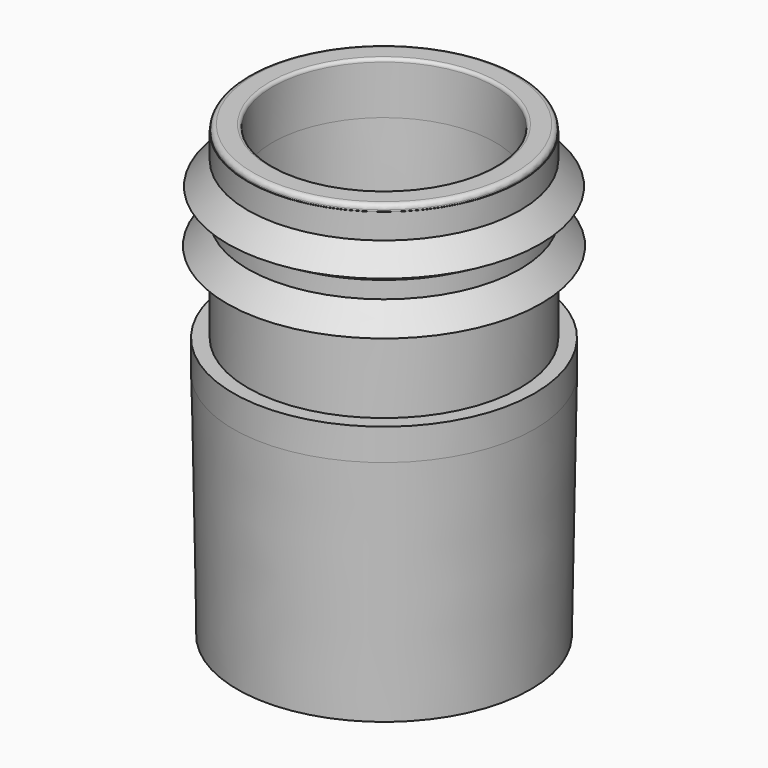
from build123d import *

# Parameters (mm, degrees)
F4_DEPTH      = 9.9510698867
F4_DEPTH_BACK = 9.9510698867


# Not quite as in the source:
# - ends of sketch curves that miss each other by under 0.0002 mm in the source are joined


with BuildPart() as f2:
    # F1 (on Front) → F2 (revolve)
    with BuildSketch(Plane.XZ):
        with BuildLine():
            Line((-0.756877, 0.003809), (-0.990799, 11.890078))
            add(Edge.make_bspline(
                [(-0.990799, 11.890078), (-0.996484, 12.183944), (-1.033002, 12.476088), (-1.099664, 12.762376)],
                knots=[0, 0, 0, 0, 1, 1, 1, 1], degree=3))
            add(Edge.make_bspline(
                [(-1.099664, 12.762376), (-1.116201, 12.833345), (-1.134632, 12.904314), (-1.154958, 12.974594)],
                knots=[0, 0, 0, 0, 1, 1, 1, 1], degree=3))
            add(Edge.make_bspline(
                [(-1.154958, 12.974594), (-1.236435, 13.256747), (-1.347022, 13.529943), (-1.485343, 13.789014)],
                knots=[0, 0, 0, 0, 1, 1, 1, 1], degree=3))
            Line((-1.485343, 13.789014), (-1.677924, 14.15006))
            Line((-1.677924, 14.15006), (-1.740797, 14.267883))
            add(Edge.make_bspline(
                [(-1.975752, 15.173254), (-1.970068, 14.856994), (-1.889625, 14.546935), (-1.740797, 14.267883)],
                knots=[0, 0, 0, 0, 1, 1, 1, 1], degree=3))
            Line((-1.975752, 15.173254), (-2.1108, 22.670126))
            Line((-2.1108, 22.670126), (-2.1108, 25.770023))
            add(Edge.make_bspline(
                [(-2.1108, 25.770023), (-2.1108, 25.88061), (-2.200372, 25.970183), (-2.310788, 25.970183)],
                knots=[0, 0, 0, 0, 1, 1, 1, 1], degree=3))
            Line((-2.310788, 25.970183), (-3.360681, 25.970183))
            add(Edge.make_bspline(
                [(-3.360681, 25.970183), (-3.52639, 25.970183), (-3.660748, 25.835824), (-3.660748, 25.670115)],
                knots=[0, 0, 0, 0, 1, 1, 1, 1], degree=3))
            Line((-3.660748, 25.670115), (-3.660748, 25.570207))
            Line((-3.660748, 25.570207), (-3.686931, 25.570207))
            Line((-3.686931, 25.570207), (-3.686931, 23.973922))
            Line((-3.686931, 23.973922), (-4.958556965, 22.5066486746))
            Line((-4.958556965, 22.5066486746), (-3.686931, 21.7700749636))
            Line((-3.686931, 21.7700749636), (-3.686931, 20.6960067153))
            Line((-3.686931, 20.6960067153), (-5.0095622428, 19.196934998))
            Line((-5.0095622428, 19.196934998), (-3.686931, 18.559782))
            Line((-3.686931, 18.559782), (-3.686931, 14.070306))
            Line((-3.686931, 14.070306), (-4.610733, 14.070306))
            Line((-4.610733, 14.070306), (-4.610733, 12.070256))
            Line((-4.610733, 12.070256), (-3.952894, -25.626775))
            ThreePointArc((-3.952894, -25.626775), (-3.2274904136, -27.9992970945), (-1.3549908614, -29.6268157026))
            Line((-1.3549908614, -29.6268157026), (1.23835, -30.835824))
            Line((1.23835, -30.835824), (1.660891, -30.929703))
            Line((1.660891, -30.929703), (2.028138, -30.929703))
            ThreePointArc((2.028138, -30.929703), (2.6539813799, -31.1498802042), (3.004306, -31.71329))
            Line((3.004306, -31.71329), (3.939132, -35.929743))
            Line((3.939132, -35.929743), (4.939071, -35.929743))
            Line((4.939071, -35.929743), (4.939243, -29.329801))
            Line((4.939243, -29.329801), (2.98553, -29.329801))
            add(Edge.make_bspline(
                [(2.732488, -29.297417), (2.814998, -29.318777), (2.900091, -29.329801), (2.98553, -29.329801)],
                knots=[0, 0, 0, 0, 1, 1, 1, 1], degree=3))
            add(Edge.make_bspline(
                [(2.67082, -29.278813), (2.691146, -29.285704), (2.711645, -29.291905), (2.732488, -29.297417)],
                knots=[0, 0, 0, 0, 1, 1, 1, 1], degree=3))
            add(Edge.make_bspline(
                [(2.44086, -29.16857), (2.512346, -29.215079), (2.589688, -29.251942), (2.67082, -29.278813)],
                knots=[0, 0, 0, 0, 1, 1, 1, 1], degree=3))
            Line((2.44086, -29.16857), (1.451946, -28.526405))
            add(Edge.make_bspline(
                [(0.087515, -26.109326), (0.119899, -27.0898), (0.629429, -27.99207), (1.451946, -28.526405)],
                knots=[0, 0, 0, 0, 1, 1, 1, 1], degree=3))
            Line((0.087515, -26.109326), (-0.686597, -2.663039))
            add(Edge.make_bspline(
                [(-0.756877, 0.003809), (-0.73948, -0.88537), (-0.716053, -1.774205), (-0.686597, -2.663039)],
                knots=[0, 0, 0, 0, 1, 1, 1, 1], degree=3))
        make_face()
    revolve(axis=Axis((4.939157, 0, -32.629772), (-2.60608e-05, 0, -0.9999999997)))

    # F3 (on Front) → F4 (cut, two sides)
    with BuildSketch(Plane.XZ) as f4_sk:
        Polygon((-27.1517578705, -2.5291696333), (-27.1517578705, -48.2453077242), (32.6887033687, -48.2453077242), (32.6887033687, -2.5307291257), align=None)
    extrude(amount=-F4_DEPTH, mode=Mode.SUBTRACT)
    extrude(f4_sk.sketch, amount=F4_DEPTH_BACK, mode=Mode.SUBTRACT)


solid = f2.part
